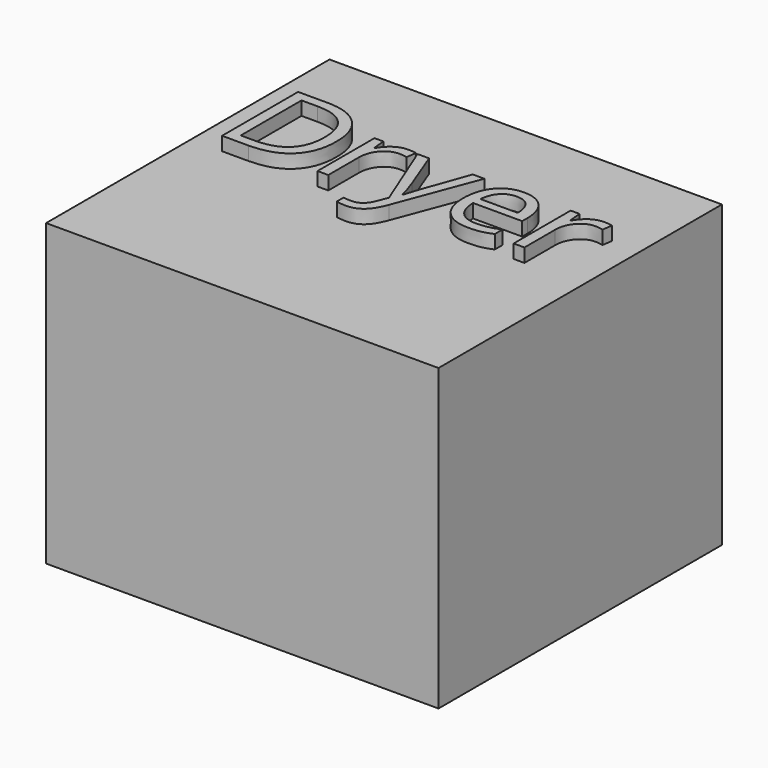
from build123d import *

# Parameters (mm, degrees)
F0_W         = 720
F0_H         = 650
F1_DEPTH     = 550
F2_TEXT_SIZE = 244.2461249413
F3_DEPTH     = 25


# Not quite as in the source:
# - Text() gives the source's letters only with a copy of the font that has no kerning and outlines rounded to 1/6400 em; it was checked with that copy


with BuildPart() as f1:
    # F0 (on Top) → F1 (new body)
    with BuildSketch(Plane.XY):
        with Locations((360, -325)):
            Rectangle(F0_W, F0_H)
    extrude(amount=F1_DEPTH)

    # F2 (on face) → F3 (join)
    with BuildSketch(Plane.XY.offset(550)):
        with Locations((33.7464878125, -318.5264638424)):
            Text('Dryer', F2_TEXT_SIZE, font='Open Sans', text_align=(TextAlign.LEFT, TextAlign.BOTTOM))
    extrude(amount=F3_DEPTH)


solid = f1.part
